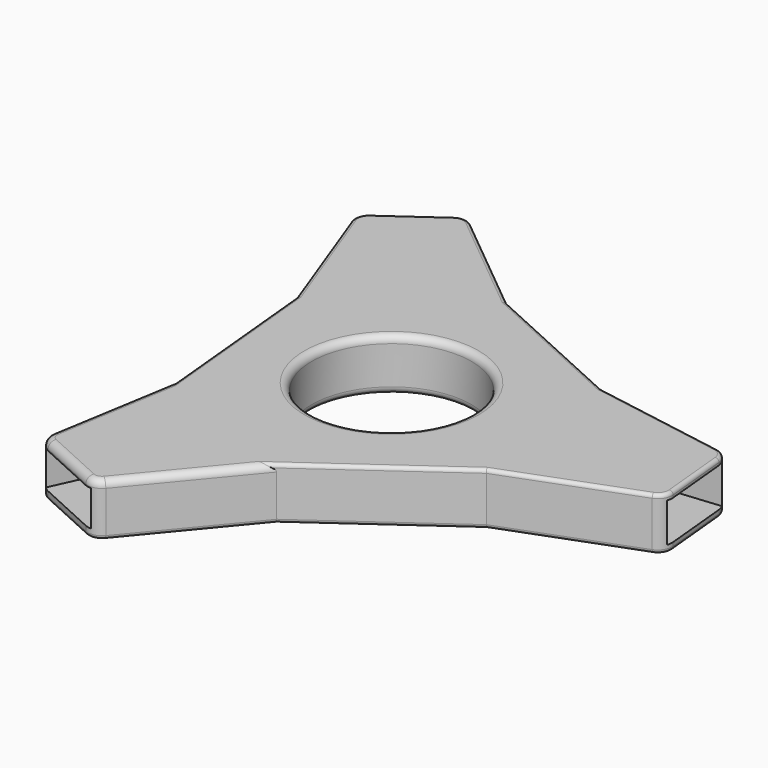
from build123d import *

# Parameters (mm, degrees)
F0_R         = 11.25
F1_DEPTH     = 2.175
F2_R         = 11.25
F3_DEPTH     = 1.5
F5_W         = 11
F5_H         = 5.5
F6_DEPTH     = 21
F7_W         = 11
F7_H         = 5.5
F8_DEPTH     = 21
F9_W         = 11
F9_H         = 5
F10_DEPTH    = 21
F11_T1_DEPTH = 15.005727874
F12_R        = 1
F13_R        = 0.5
F14_R        = 0.5
F15_R        = 0.5
F16_R        = 0.5
F17_R        = 0.5
F18_R        = 0.5
F19_R        = 0.5
F20_R        = 1


# Not quite as in the source:
# - a fillet or chamfer that OpenCascade refuses, or shapes differently, is made with other operations: its cross-section is extruded or revolved along the edge and cut away or added


with BuildPart() as f1:
    # F0 (on Top) → F1 (new body, symmetric)
    with BuildSketch(Plane.XY):
        Polygon((-2.2081266769, 22.9882037122), (-21.0124317406, 9.5818080591), (-18.8043050636, -13.4063956531), (2.2081266769, -22.9882037122), (21.0124317406, -9.5818080591), (18.8043050636, 13.4063956531), align=None)
        Circle(F0_R, mode=Mode.SUBTRACT)
        Polygon((-28.2205584175, 29.0052973062), (-21.0124317406, 9.5818080591), (-2.2081266769, 22.9882037122), (-18.2205584175, 36.1347262363), align=None)
        Polygon((2.2081266769, -22.9882037122), (-18.8043050636, -13.4063956531), (-22.1833116707, -33.8468295789), (-11.0090451027, -38.9423691517), align=None)
        Polygon((39.2296035202, 9.9370718455), (18.8043050636, 13.4063956531), (21.0124317406, -9.5818080591), (40.4038700882, -2.2878966574), align=None)
    extrude(amount=F1_DEPTH, both=True)

    # F2 (on face) → F3 (join)
    with BuildSketch(Plane.XY.offset(2.175)):
        Polygon((-18.8043050636, -13.4063956531), (-22.1833116707, -33.8468295789), (-11.0090451027, -38.9423691517), (2.2081266769, -22.9882037122), (21.0124317406, -9.5818080591), (40.4038700882, -2.2878966574), (39.2296035202, 9.9370718455), (18.8043050636, 13.4063956531), (-2.2081266769, 22.9882037122), (-18.2205584175, 36.1347262363), (-28.2205584175, 29.0052973062), (-21.0124317406, 9.5818080591), align=None)
        Circle(F2_R, mode=Mode.SUBTRACT)
    extrude(amount=F3_DEPTH)

    # F4: F1 across plane


with BuildPart() as f1_1:
    add(f1.part)
    add(f1.part.mirror(Plane.XY))

    # F5 (on face) → F6 (cut)
    with BuildSketch(Plane(origin=(39.8167368042, 3.824587594, 0), x_dir=(-0.0956146899, 0.9954184201, 0), z_dir=(0.9954184201, 0.0956146899, 0))):
        with Locations((0.0001179833, 0.075)):
            Rectangle(F5_W, F5_H)
    extrude(amount=-F6_DEPTH, mode=Mode.SUBTRACT)

    # F7 (on face) → F8 (cut)
    with BuildSketch(Plane(origin=(-23.2205584175, 32.5700117712, 0), x_dir=(-0.8142502943, -0.5805139604, 0), z_dir=(-0.5805139604, 0.8142502943, 0))):
        with Locations((0.0003820167, 0)):
            Rectangle(F7_W, F7_H)
    extrude(amount=-F8_DEPTH, mode=Mode.SUBTRACT)

    # F9 (on face) → F10 (cut)
    with BuildSketch(Plane(origin=(-16.5961783867, -36.3945993653, 0), x_dir=(0.9098649841, -0.4149044597, 0), z_dir=(-0.4149044597, -0.9098649841, 0))):
        with Locations((0.0001179833, 0)):
            Rectangle(F9_W, F9_H)
    extrude(amount=-F10_DEPTH, mode=Mode.SUBTRACT)

    # F11: fillet of radius 2 on 6 edges, made by hand

    # F11_s2 → F11_t1 (cut)
    with BuildSketch(Plane.XY.offset(-7.502863937)):
        with BuildLine():
            ThreePointArc((-17.0371647686, 35.1631366918), (-18.2382120361, 35.6162160874), (-19.4672941524, 35.2458748546))
            Line((-19.4672941524, 35.2458748546), (-18.2205584175, 36.1347262363))
            Line((-18.2205584175, 36.1347262363), (-17.0371647686, 35.1631366918))
        make_face()
        with BuildLine():
            ThreePointArc((-27.6878441198, 27.5698105427), (-27.7246206597, 28.8529484789), (-26.9738226827, 29.8941486878))
            Line((-26.9738226827, 29.8941486878), (-28.2205584175, 29.0052973062))
            Line((-28.2205584175, 29.0052973062), (-27.6878441198, 27.5698105427))
        make_face()
        with BuildLine():
            ThreePointArc((-21.9335872676, -32.336185844), (-21.7254419003, -33.6028629865), (-20.7901759265, -34.4821087062))
            Line((-20.7901759265, -34.4821087062), (-22.1833116707, -33.8468295789))
            Line((-22.1833116707, -33.8468295789), (-21.9335872676, -32.336185844))
        make_face()
        with BuildLine():
            ThreePointArc((-12.4021808468, -38.3070900243), (-11.125076027, -38.4367000411), (-10.0322342476, -37.7632816551))
            Line((-10.0322342476, -37.7632816551), (-11.0090451027, -38.9423691517))
            Line((-11.0090451027, -38.9423691517), (-12.4021808468, -38.3070900243))
        make_face()
        with BuildLine():
            ThreePointArc((38.9707520362, -2.8269508478), (39.9636539364, -2.0133531008), (40.2574700789, -0.7637661484))
            Line((40.2574700789, -0.7637661484), (40.4038700882, -2.2878966574))
            Line((40.4038700882, -2.2878966574), (38.9707520362, -2.8269508478))
        make_face()
        with BuildLine():
            ThreePointArc((37.7200783674, 10.1934711124), (38.8496966867, 9.5837515621), (39.3760035295, 8.4129413364))
            Line((39.3760035295, 8.4129413364), (39.2296035202, 9.9370718455))
            Line((39.2296035202, 9.9370718455), (37.7200783674, 10.1934711124))
        make_face()
    extrude(amount=F11_T1_DEPTH, mode=Mode.SUBTRACT)

    # F12
    f12_edges = [f1_1.edges().sort_by_distance(p)[0] for p in [
        (-16.596178, -36.394599, 3.675),
    ]]
    fillet(f12_edges, radius=F12_R)

    # F13
    f13_edges = [f1_1.edges().sort_by_distance(p)[0] for p in [
        (29.991592, -6.204379, 3.675),
    ]]
    fillet(f13_edges, radius=F13_R)

    # F14
    f14_edges = [f1_1.edges().sort_by_distance(p)[0] for p in [
        (-23.220558, 32.570012, 3.675),
    ]]
    fillet(f14_edges, radius=F14_R)

    # F15
    f15_edges = [f1_1.edges().sort_by_distance(p)[0] for p in [
        (-19.908368, -1.912294, 3.675),
        (11.610279, -16.285006, 3.675),
        (8.298089, 18.1973, 3.675),
    ]]
    fillet(f15_edges, radius=F15_R)

    # F16
    f16_edges = [f1_1.edges().sort_by_distance(p)[0] for p in [
        (-24.350138, 18.575809, -3.675),
    ]]
    fillet(f16_edges, radius=F16_R)

    # F17
    f17_edges = [f1_1.edges().sort_by_distance(p)[0] for p in [
        (28.262192, 11.799933, -3.675),
    ]]
    fillet(f17_edges, radius=F17_R)

    # F18
    f18_edges = [f1_1.edges().sort_by_distance(p)[0] for p in [
        (-3.912054, -30.375743, -3.675),
    ]]
    fillet(f18_edges, radius=F18_R)

    # F19
    f19_edges = [f1_1.edges().sort_by_distance(p)[0] for p in [
        (-19.908368, -1.912294, -3.675),
        (11.610279, -16.285006, -3.675),
        (8.298089, 18.1973, -3.675),
    ]]
    fillet(f19_edges, radius=F19_R)

    # F20
    f20_edges = [f1_1.edges().sort_by_distance(p)[0] for p in [
        (-11.25, 0, 3.675),
        (-11.25, 0, -3.675),
    ]]
    fillet(f20_edges, radius=F20_R)


solid = f1_1.part
